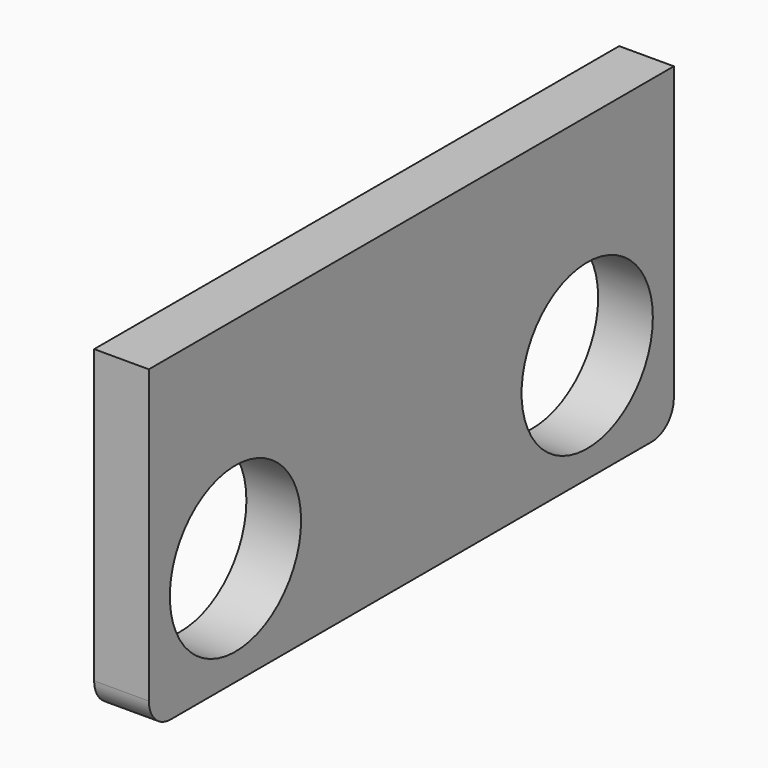
from build123d import *

# Parameters (mm, degrees)
F0_W     = 13.5
F0_H     = 6.75
F1_DEPTH = 20
F2_W     = 8
F2_H     = 26.4694701647
F3_DEPTH = 12
F4_R     = 0.49999
F7_R     = 7.5
F8_DEPTH = 5
F9_T     = -2


# Not quite as in the source:
# - a fillet or chamfer is up to 0.001 mm smaller than in the source, because OpenCascade refuses the exact size
# - a feature of the source that left no trace in its solid (it failed there, or was rolled back) is left out


with BuildPart() as f1:
    # F0 (on Right) → F1 (new body)
    with BuildSketch(Plane.YZ):
        with BuildLine():
            Line((21.2005410668, -21.2570374378), (21.2005410668, 3.4429625622))
            Line((21.2005410668, 3.4429625622), (24.7505410668, 3.4429625622))
            Line((24.7505410668, 3.4429625622), (24.7505410668, -5.3425713437))
            Line((24.7505410668, -5.3425713437), (24.7505410668, -14.0570374378))
            ThreePointArc((24.7505410668, -14.0570374378), (25.4827741138, -15.8248043907), (27.2505410668, -16.5570374378))
            Line((27.2505410668, -16.5570374378), (31.4505410668, -16.5570374378))
            ThreePointArc((31.4505410668, -16.5570374378), (33.2183080197, -15.8248043907), (33.9505410668, -14.0570374378))
            Line((33.9505410668, -14.0570374378), (33.9505410668, -5.3425713437))
            Line((33.9505410668, -5.3425713437), (33.9505410668, 6.3718947504))
            ThreePointArc((33.9505410668, 6.3718947504), (34.4092996144, 7.8152704233), (35.6172077334, 8.7289173543))
            ThreePointArc((35.6172077334, 8.7289173543), (37.4860749727, 16.9784964681), (29.2364958588, 15.1096292289))
            ThreePointArc((29.2364958588, 15.1096292289), (28.3228489279, 13.9017211099), (26.8794732549, 13.4429625622))
            Line((26.8794732549, 13.4429625622), (15.2005410668, 13.4429625622))
            Line((15.2005410668, 13.4429625622), (-1.2994589332, 13.4429625622))
            ThreePointArc((-1.2994589332, 13.4429625622), (-3.0672258862, 12.7107295152), (-3.7994589332, 10.9429625622))
            Line((-3.7994589332, 10.9429625622), (-3.7994589332, 5.9429625622))
            ThreePointArc((-3.7994589332, 5.9429625622), (-3.0672258862, 4.1751956093), (-1.2994589332, 3.4429625622))
            Line((-1.2994589332, 3.4429625622), (5.1650071608, 3.4429625622))
            ThreePointArc((5.1650071608, 3.4429625622), (6.1217157417, 3.2526613935), (6.9327741138, 2.7107295152))
            Line((6.9327741138, 2.7107295152), (14.4934342856, -4.8499306566))
            Line((14.4934342856, -4.8499306566), (15.4683080197, -5.8248043907))
            ThreePointArc((15.4683080197, -5.8248043907), (16.010239898, -6.6358627628), (16.2005410668, -7.5925713437))
            Line((16.2005410668, -7.5925713437), (16.2005410668, -21.2570374378))
            ThreePointArc((16.2005410668, -21.2570374378), (16.4934342856, -21.964144219), (17.2005410668, -22.2570374378))
            Line((17.2005410668, -22.2570374378), (20.2005410668, -22.2570374378))
            ThreePointArc((20.2005410668, -22.2570374378), (20.9076478479, -21.964144219), (21.2005410668, -21.2570374378))
        make_face()
        with Locations((5.7005410668, 7.8179625622)):
            Rectangle(F0_W, F0_H, mode=Mode.SUBTRACT)
    extrude(amount=F1_DEPTH)

    # F2 (on face) → F3 (cut)
    with BuildSketch(Plane.YZ.offset(20)):
        with Locations((5.7005410668, 11.1929625622)):
            Rectangle(F2_W, F2_H)
    extrude(amount=-F3_DEPTH, mode=Mode.SUBTRACT)

    # F4 (radius 0.5 in the source; OpenCascade refuses exactly that, so slightly less here)
    f4_edges = [f1.edges().sort_by_distance(p)[0] for p in [
        (14, 1.700541, 11.192963),
        (14, 1.700541, 13.442963),
        (14, 1.700541, 4.442963),
        (14, 1.700541, 3.442963),
        (10, -1.049459, 4.442963),
        (10, -1.049459, 11.192963),
        (10, 12.450541, 11.192963),
        (10, 12.450541, 4.442963),
        (14, 9.700541, 11.192963),
        (14, 9.700541, 13.442963),
        (14, 9.700541, 4.442963),
    ]]
    fillet(f4_edges, radius=F4_R)


with BuildPart() as f8:
    # F7 (on Right) → F8 (new body)
    with BuildSketch(Plane.YZ):
        with BuildLine():
            Line((-17.6103499532, 45.065652512), (-22.6103499532, 45.065652512))
            Line((-22.6103499532, 45.065652512), (-72.6103499532, 45.065652512))
            Line((-72.6103499532, 45.065652512), (-77.6103499532, 45.065652512))
            Line((-77.6103499532, 45.065652512), (-77.6103499532, 27.565652512))
            ThreePointArc((-77.6103499532, 27.565652512), (-76.8781169061, 25.7978855591), (-75.1103499532, 25.065652512))
            Line((-75.1103499532, 25.065652512), (-20.1103499532, 25.065652512))
            ThreePointArc((-20.1103499532, 25.065652512), (-18.3425830002, 25.7978855591), (-17.6103499532, 27.565652512))
            Line((-17.6103499532, 27.565652512), (-17.6103499532, 45.065652512))
        make_face()
        with Locations((-67.7103499532, 35.015652512)):
            Circle(F7_R, mode=Mode.SUBTRACT)
        with Locations((-27.5103499532, 35.015652512)):
            Circle(F7_R, mode=Mode.SUBTRACT)
        Polygon((-72.6103499532, 45.065652512), (-22.6103499532, 45.065652512), (-17.6103499532, 45.065652512), (-17.6103499532, 54.265652512), (-77.6103499532, 54.265652512), (-77.6103499532, 45.065652512), align=None)
    extrude(amount=F8_DEPTH)

    # F9
    f9_openings = [f8.faces().sort_by_distance(p)[0] for p in [
        (0, -47.61035, 40.869984),
    ]]
    offset(amount=F9_T, openings=f9_openings)


solid = f8.part
